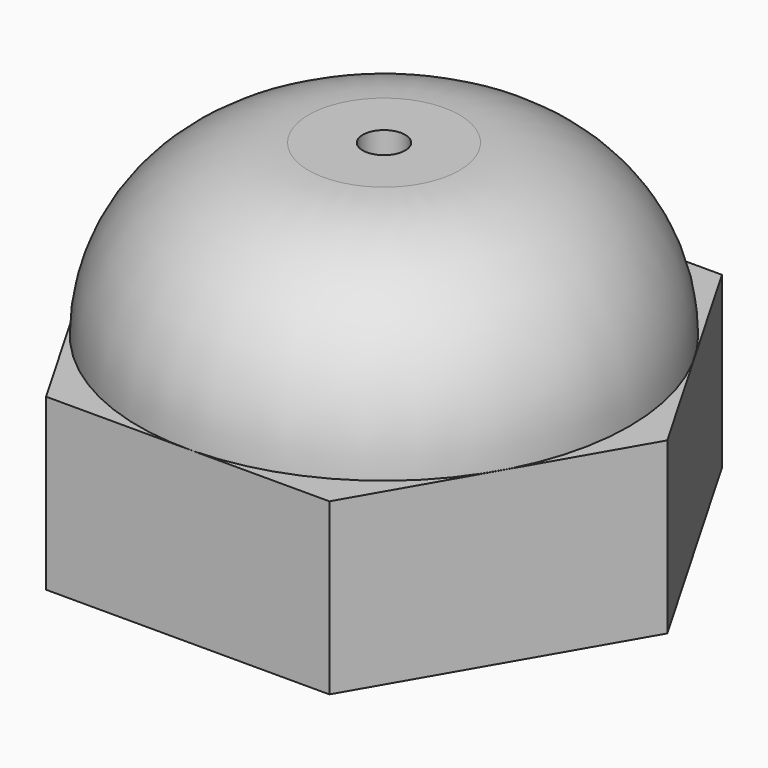
from build123d import *

# Parameters (mm, degrees)
F0_R     = 3.5
F1_DEPTH = 6
F2_R     = 8.6602540378
F3_DEPTH = 6
F4_R     = 5.99999
F6_DEPTH = 3
F5_R     = 0.75
F7_DEPTH = 12.001


# Not quite as in the source:
# - a fillet or chamfer is up to 0.001 mm smaller than in the source, because OpenCascade refuses the exact size


with BuildPart() as f1:
    # F0 (on Top) → F1 (new body)
    with BuildSketch(Plane.XY):
        Polygon((5, 8.6602540378), (-5, 8.6602540378), (-10, 0), (-5, -8.6602540378), (5, -8.6602540378), (10, 0), align=None)
        Circle(F0_R, mode=Mode.SUBTRACT)
    extrude(amount=F1_DEPTH)

    # F2 (on face) → F3 (join)
    with BuildSketch(Plane.XY.offset(6)):
        Circle(F2_R)
    extrude(amount=F3_DEPTH)

    # F4 (radius 6 in the source; OpenCascade refuses exactly that, so slightly less here)
    f4_edges = [f1.edges().sort_by_distance(p)[0] for p in [
        (-8.660254, 0, 12),
    ]]
    fillet(f4_edges, radius=F4_R)

    # F6 (cut): a face of the model
    f6_faces = [f1.faces().sort_by_distance(p)[0] for p in [
        (0, 0, 6),
    ]]
    extrude(f6_faces, amount=-F6_DEPTH, mode=Mode.SUBTRACT)

    # F5 (on face) → F7 (cut, through all)
    with BuildSketch(Plane.XY.offset(12)):
        Circle(F5_R)
    extrude(amount=-F7_DEPTH, mode=Mode.SUBTRACT)


solid = f1.part
